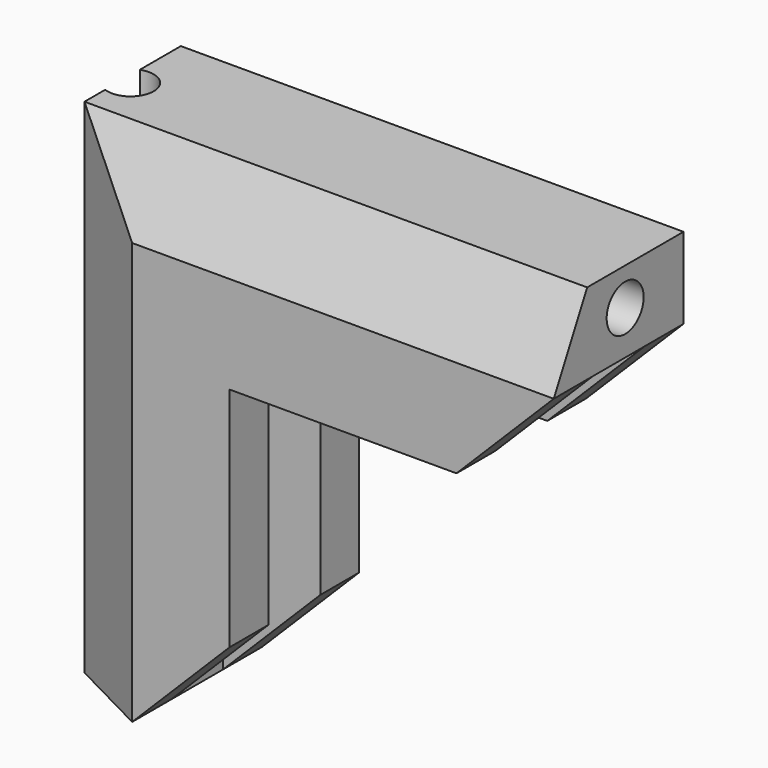
from build123d import *

# Parameters (mm, degrees)
F1_DEPTH      = 20
F2_W          = 7
F2_H          = 20
F3_DEPTH      = 2
F5_DEPTH      = 6
F6_W          = 3
F6_H          = 6
F7_DEPTH      = 25
F8_DEPTH      = 3
F12_DEPTH     = 2
F13_DEPTH     = 11
F14_T4_DEPTH  = 29
F14_T10_DEPTH = 28
F14_T17_DEPTH = 38.2867319519
F14_T24_DEPTH = 39.2867319519
F15_T1_DEPTH  = 61.1449358039
F15_T3_DEPTH  = 60.1449358039
F16_DEPTH     = 1
F17_SIZE      = 6
F20_D         = 2.85
F20_ON_F18_D  = 2.85


# Not quite as in the source:
# - a fillet or chamfer that OpenCascade refuses, or shapes differently, is made with other operations: its cross-section is extruded or revolved along the edge and cut away or added


with BuildPart() as f1:
    # F0 (on Top) → F1 (new body)
    with BuildSketch(Plane.XY):
        Polygon((-3.1551690071, 9.1141472052), (-12.1551690071, 9.1141472052), (-12.1551690071, -0.8858527948), (-3.1551690071, -0.8858527948), (-3.1551690071, 2.1141472052), (-9.1551690071, 2.1141472052), (-9.1551690071, 6.1141472052), (-3.1551690071, 6.1141472052), align=None)
    extrude(amount=F1_DEPTH)

    # F2 (on face) → F3 (join)
    with BuildSketch(Plane(origin=(-12.1551690071, 0, 0), x_dir=(0, -1, 0), z_dir=(-1, 0, 0))):
        with Locations((-5.6141472052, 10)):
            Rectangle(F2_W, F2_H)
    extrude(amount=F3_DEPTH)

    # F4 (on face) → F5 (join)
    with BuildSketch(Plane.XY.offset(20)):
        Polygon((-12.1345976368, 9.1141472052), (-12.1551690071, 2.1141472052), (-12.1551690071, -0.8858527948), (-9.1551690071, -0.8858527948), (-9.1551690071, 2.1141472052), (-9.1551690071, 6.1141472052), (-9.1551690071, 9.1141472052), align=None)
    extrude(amount=F5_DEPTH)

    # F6 (on face) → F7 (join)
    with BuildSketch(Plane.YZ.offset(-9.1551690071)):
        with Locations((7.6141472052, 23)):
            Rectangle(F6_W, F6_H)
        with Locations((0.6141472052, 23)):
            Rectangle(F6_W, F6_H)
        Polygon((-0.8858527948, 26), (2.1141472052, 26), (6.1141472052, 26), (9.1141472052, 26), (9.1141472052, 29), (-0.8858527948, 29), align=None)
    extrude(amount=F7_DEPTH)

    # F8 (add): a face of the model
    f8_faces = [f1.faces().sort_by_distance(p)[0] for p in [
        (-10.6515768532, 4.1077318265, 26),
    ]]
    extrude(f8_faces, amount=F8_DEPTH)

    # F9: union 

    # F10: union 

    # F11 (on face) → F12 (join)
    with BuildSketch(Plane.XY.offset(29)):
        Polygon((-12.1345976368, 9.1141472052), (-12.1551690071, 2.1141472052), (15.8448309929, 2.1141472052), (15.8448309929, 9.1141472052), align=None)
    extrude(amount=F12_DEPTH)

    # F4 (on face) → F13 (join)
    with BuildSketch(Plane.XY.offset(20)):
        Polygon((-14.1551690071, 2.1141472052), (-12.1551690071, 2.1141472052), (-12.1345976368, 9.1141472052), (-14.1551690071, 9.1141472052), align=None)
    extrude(amount=F13_DEPTH)

    # F14: chamfer of 4 on 2 edges, made by hand


with BuildPart() as f14_tool2:
    # F14_s3 → F14_t4 (new body)
    with BuildSketch(Plane.XY):
        Polygon((-12.1551690071, -1.8858527948), (-16.1551690071, 2.1141472052), (-12.1551690071, 2.1141472052), align=None)
    extrude(amount=F14_T4_DEPTH)

    split(bisect_by=Plane.XZ.offset(0.8858527948), keep=Keep.BOTTOM)

    split(bisect_by=Plane.YZ.offset(-14.1551690071), keep=Keep.TOP)


with BuildPart() as f1_1:
    add(f1.part)

    # F14_t1: union F14_tool2
    add(f14_tool2.part)


with BuildPart() as f14_tool8:
    # F14_s9 → F14_t10 (new body)
    with BuildSketch(Plane.YZ.offset(-12.1551690071)):
        Polygon((-1.8858527948, 29), (2.1141472052, 33), (2.1141472052, 29), align=None)
    extrude(amount=F14_T10_DEPTH)

    split(bisect_by=Plane.XZ.offset(0.8858527948), keep=Keep.BOTTOM)

    split(bisect_by=Plane.XY.offset(31), keep=Keep.BOTTOM)


with BuildPart() as f1_2:
    add(f1_1.part)

    # F14_t7: union F14_tool8
    add(f14_tool8.part)


with BuildPart() as f14_tool15:
    # F14_s16 → F14_t17 (new body)
    with BuildSketch(Plane.YZ.offset(-22.4419009589)):
        Polygon((-1.8858527948, 29), (2.1141472052, 33), (2.1141472052, 29), align=None)
    extrude(amount=F14_T17_DEPTH)

    split(bisect_by=Plane.XZ.offset(0.8858527948), keep=Keep.BOTTOM)

    split(bisect_by=Plane.YZ.offset(-12.1551690071), keep=Keep.BOTTOM)

    split(bisect_by=Plane.YZ.offset(-14.1551690071), keep=Keep.TOP)

    split(bisect_by=Plane.XY.offset(31), keep=Keep.BOTTOM)


with BuildPart() as f14_tool22:
    # F14_s23 → F14_t24 (new body)
    with BuildSketch(Plane.XY):
        Polygon((-12.1551690071, -1.8858527948), (-16.1551690071, 2.1141472052), (-12.1551690071, 2.1141472052), align=None)
    extrude(amount=F14_T24_DEPTH)

    split(bisect_by=Plane.XZ.offset(0.8858527948), keep=Keep.BOTTOM)

    split(bisect_by=Plane.XY.offset(29), keep=Keep.TOP)

    split(bisect_by=Plane.YZ.offset(-14.1551690071), keep=Keep.TOP)

    split(bisect_by=Plane.XY.offset(31), keep=Keep.BOTTOM)


with BuildPart() as f14_tool15_1:
    add(f14_tool15.part)

    # F14_t29: intersect F14_tool22
    add(f14_tool22.part, mode=Mode.INTERSECT)


with BuildPart() as f1_3:
    add(f1_2.part)

    # F14_t13: union F14_tool15
    add(f14_tool15_1.part)

    # F15: chamfer of 4 x 6 on 2 edges, made by hand

    # F15_s2 → F15_t1 (cut)
    with BuildSketch(Plane.XY.offset(-15.5724679019)):
        Polygon((-9.1551690071, -0.8858527948), (-17.3978096942, 3.3567878923), (-13.1551690071, -0.8858527948), align=None)
    extrude(amount=F15_T1_DEPTH, mode=Mode.SUBTRACT)

    # F15_s4 → F15_t3 (cut)
    with BuildSketch(Plane.YZ.offset(-28.7276369091)):
        Polygon((-0.8858527948, 26), (3.3567878923, 34.2426406871), (-0.8858527948, 30), align=None)
    extrude(amount=F15_T3_DEPTH, mode=Mode.SUBTRACT)

    # F16 (add): a face of the model
    f16_faces = [f1_3.faces().sort_by_distance(p)[0] for p in [
        (15.8448309929, 6.2628078927, 23),
    ]]
    extrude(f16_faces, amount=F16_DEPTH)

    # F17
    f17_edges = [f1_3.edges().sort_by_distance(p)[0] for p in [
        (-3.155169, 0.614147, 0),
        (-3.155169, 7.614147, 0),
        (16.844831, 0.614147, 20),
        (16.844831, 7.614147, 20),
    ]]
    chamfer(f17_edges, length=F17_SIZE)

    # F20 (through all)
    with Locations(Plane(origin=(0, 0, 0), x_dir=(1, 0, 0), z_dir=(0, 0, -1))):
        with Locations((-13.6551690071, -4.6141472052)):
            Hole(F20_D / 2)

    # F20 on F18 (through all)
    with Locations(Plane.YZ.offset(16.8448309929)):
        with Locations((4.6141472052, 28.7)):
            Hole(F20_ON_F18_D / 2)


solid = f1_3.part
